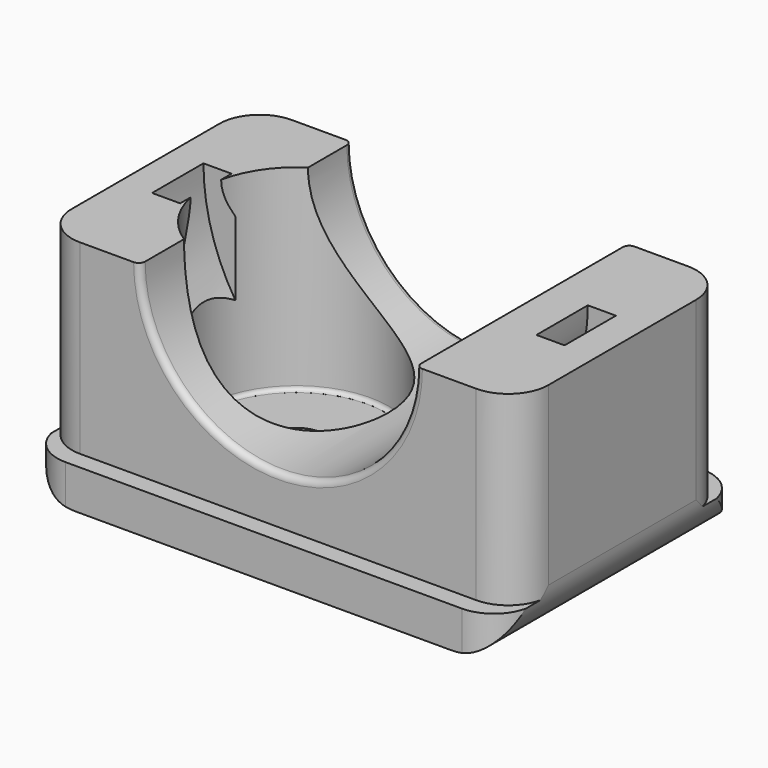
from build123d import *

# Parameters (mm, degrees)
F2_W         = 30.1625
F2_H         = 19.05
F2_R         = 5.842
F2_R_2       = 1.8161
F3_DEPTH     = 2.54
F5_DEPTH     = 2.032
F7_DEPTH     = 6.35
F8_DEPTH     = 2.032
F9_DEPTH     = 2.032
F11_DEPTH    = 14.32025
F12_R        = 5.842
F13_DEPTH    = 12.41425
F14_R        = 2.54
F15_R        = 0.4064
F16_R        = 0.254
F17_T1_DEPTH = 18.2149387894
F18_T1_DEPTH = 29.845


# Not quite as in the source:
# - a fillet or chamfer that OpenCascade refuses, or shapes differently, is made with other operations: its cross-section is extruded or revolved along the edge and cut away or added


with BuildPart() as f3:
    # F2 (on Top) → F3 (new body)
    with BuildSketch(Plane.XY):
        with Locations((5.55625, 0)):
            Rectangle(F2_W, F2_H)
        Circle(F2_R, mode=Mode.SUBTRACT)
        Circle(F2_R)
        Circle(F2_R_2, mode=Mode.SUBTRACT)
    extrude(amount=F3_DEPTH)

    # F4 (on Front) → F5 (join, symmetric)
    with BuildSketch(Plane.XZ):
        with BuildLine():
            ThreePointArc((1.5351403895, 1.905), (-4.9973131459, 6.6442757011), (-7.493, 14.31925))
            Line((-7.493, 14.31925), (-9.525, 14.31925))
            Line((-9.525, 14.31925), (-9.525, 0))
            Line((-9.525, 0), (20.6375, 0))
            Line((20.6375, 0), (20.6375, 14.31925))
            Line((20.6375, 14.31925), (18.6055, 14.31925))
            ThreePointArc((18.6055, 14.31925), (16.1098131459, 6.6442757011), (9.5773596105, 1.905))
            Line((9.5773596105, 1.905), (1.5351403895, 1.905))
        make_face()
    extrude(amount=F5_DEPTH, both=True)

    # F6 (on face) → F7 (join)
    with BuildSketch(Plane.XZ.offset(2.032)):
        with BuildLine():
            Line((-3.175, 14.31925), (-9.525, 14.31925))
            Line((-9.525, 14.31925), (-9.525, 0))
            Line((-9.525, 0), (20.6375, 0))
            Line((20.6375, 0), (20.6375, 14.31925))
            Line((20.6375, 14.31925), (14.2875, 14.31925))
            ThreePointArc((14.2875, 14.31925), (5.55625, 5.588), (-3.175, 14.31925))
        make_face()
    extrude(amount=F7_DEPTH)

    # F4 (on Front) → F8 (cut, symmetric)
    with BuildSketch(Plane.XZ):
        with BuildLine():
            ThreePointArc((0.3585509899, 4.318), (-4.0776910817, 8.4687580722), (-5.715, 14.31925))
            Line((-5.715, 14.31925), (-7.493, 14.31925))
            ThreePointArc((-7.493, 14.31925), (-4.9973131459, 6.6442757011), (1.5351403895, 1.905))
            Line((1.5351403895, 1.905), (9.5773596105, 1.905))
            ThreePointArc((9.5773596105, 1.905), (16.1098131459, 6.6442757011), (18.6055, 14.31925))
            Line((18.6055, 14.31925), (16.8275, 14.31925))
            ThreePointArc((16.8275, 14.31925), (15.1901910817, 8.4687580722), (10.7539490101, 4.318))
            Line((10.7539490101, 4.318), (0.3585509899, 4.318))
        make_face()
    extrude(amount=F8_DEPTH, both=True, mode=Mode.SUBTRACT)

    # F4 (on Front) → F9 (join, through all)
    with BuildSketch(Plane.XZ):
        with BuildLine():
            ThreePointArc((14.2875, 14.31925), (5.55625, 5.588), (-3.175, 14.31925))
            Line((-3.175, 14.31925), (-5.715, 14.31925))
            ThreePointArc((-5.715, 14.31925), (-4.0776910817, 8.4687580722), (0.3585509899, 4.318))
            Line((0.3585509899, 4.318), (10.7539490101, 4.318))
            ThreePointArc((10.7539490101, 4.318), (15.1901910817, 8.4687580722), (16.8275, 14.31925))
            Line((16.8275, 14.31925), (14.2875, 14.31925))
        make_face()
    extrude(amount=F9_DEPTH)

    # F10: F3 across plane


with BuildPart() as f3_1:
    add(f3.part)
    add(f3.part.mirror(Plane.XZ))

    # F2 (on Top) → F11 (cut, through all)
    with BuildSketch(Plane.XY):
        Circle(F2_R_2)
    extrude(amount=F11_DEPTH, mode=Mode.SUBTRACT)

    # F12 (on face) → F13 (cut, through all)
    with BuildSketch(Plane.XY.offset(14.31925)):
        Circle(F12_R)
    extrude(amount=-F13_DEPTH, mode=Mode.SUBTRACT)

    # F14
    f14_edges = [f3_1.edges().sort_by_distance(p)[0] for p in [
        (20.6375, 9.525, 1.27),
        (-9.525, 9.525, 1.27),
        (20.6375, -9.525, 1.27),
        (-9.525, -9.525, 1.27),
    ]]
    fillet(f14_edges, radius=F14_R)

    # F15
    f15_edges = [f3_1.edges().sort_by_distance(p)[0] for p in [
        (5.55625, -8.382, 5.588),
        (5.55625, 8.382, 5.588),
    ]]
    fillet(f15_edges, radius=F15_R)

    # F16
    f16_edges = [f3_1.edges().sort_by_distance(p)[0] for p in [
        (-5.842, 0, 1.905),
    ]]
    fillet(f16_edges, radius=F16_R)

    # F17: fillet of radius 2.54 on 4 edges, made by hand

    # F17_s2 → F17_t1 (cut)
    with BuildSketch(Plane.XY.offset(2.54)):
        with BuildLine():
            ThreePointArc((-6.985, -8.382), (-8.7810512242, -7.6380512242), (-9.525, -5.842))
            Line((-9.525, -5.842), (-9.779, -5.842))
            ThreePointArc((-9.779, -5.842), (-9.779, -6.985), (-9.3184500445, -8.5217))
            Line((-9.3184500445, -8.5217), (-9.1063182222, -8.636))
            Line((-9.1063182222, -8.636), (-6.985, -8.636))
            Line((-6.985, -8.636), (-6.985, -8.382))
        make_face()
        with BuildLine():
            ThreePointArc((18.0975, -8.382), (19.8935512242, -7.6380512242), (20.6375, -5.842))
            Line((20.6375, -5.842), (20.8915, -5.842))
            ThreePointArc((20.8915, -5.842), (20.8915, -6.985), (20.4309500445, -8.5217))
            Line((20.4309500445, -8.5217), (20.2188182222, -8.636))
            Line((20.2188182222, -8.636), (18.0975, -8.636))
            Line((18.0975, -8.636), (18.0975, -8.382))
        make_face()
        with BuildLine():
            ThreePointArc((20.6375, 5.842), (19.8935512242, 7.6380512242), (18.0975, 8.382))
            Line((18.0975, 8.382), (18.0975, 8.636))
            Line((18.0975, 8.636), (20.2188182222, 8.636))
            Line((20.2188182222, 8.636), (20.4309500445, 8.5217))
            ThreePointArc((20.4309500445, 8.5217), (20.8915, 6.985), (20.8915, 5.842))
            Line((20.8915, 5.842), (20.6375, 5.842))
        make_face()
        with BuildLine():
            ThreePointArc((-6.985, 8.382), (-8.7810512242, 7.6380512242), (-9.525, 5.842))
            Line((-9.525, 5.842), (-9.779, 5.842))
            ThreePointArc((-9.779, 5.842), (-9.779, 6.985), (-9.3184500445, 8.5217))
            Line((-9.3184500445, 8.5217), (-9.1063182222, 8.636))
            Line((-9.1063182222, 8.636), (-6.985, 8.636))
            Line((-6.985, 8.636), (-6.985, 8.382))
        make_face()
    extrude(amount=F17_T1_DEPTH, mode=Mode.SUBTRACT)

    # F18: fillet of radius 3.175 on 2 edges, made by hand

    # F18_s2 → F18_t1 (cut)
    with BuildSketch(Plane.XZ.offset(-14.9225)):
        with BuildLine():
            ThreePointArc((17.4625, 0), (19.7075640303, 0.9299359697), (20.6375, 3.175))
            Line((20.6375, 3.175), (20.6375, 0))
            Line((20.6375, 0), (17.4625, 0))
        make_face()
        with BuildLine():
            ThreePointArc((-9.525, 3.175), (-8.5950640303, 0.9299359697), (-6.35, 0))
            Line((-6.35, 0), (-9.525, 0))
            Line((-9.525, 0), (-9.525, 3.175))
        make_face()
    extrude(amount=F18_T1_DEPTH, mode=Mode.SUBTRACT)


solid = f3_1.part
